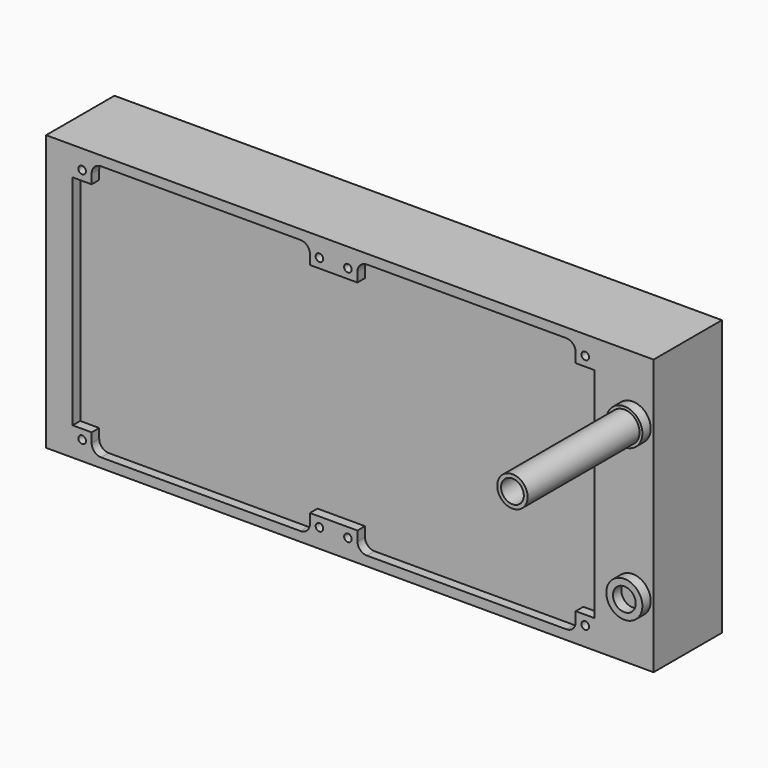
from build123d import *

# Parameters (mm, degrees)
F0_W     = 320
F0_H     = 145
F1_DEPTH = 45
F2_R     = 9.5
F2_R_2   = 6
F3_DEPTH = 5.5
F4_R     = 2
F5_DEPTH = 5
F7_R     = 8
F7_R_2   = 6
F8_DEPTH = 73.6875


# Not quite as in the source:
# - a pattern or mirror of a feature is missing from the dataset's text; its kind, count and spacing are read off the source's solid


with BuildPart() as f1:
    # F0 (on Front) → F1 (new body)
    with BuildSketch(Plane.XZ):
        with Locations((160, 0)):
            Rectangle(F0_W, F0_H)
    extrude(amount=F1_DEPTH)

    # F2 (on face) → F3 (join)
    with BuildSketch(Plane.XZ.offset(45)):
        with Locations((309, -40)):
            Circle(F2_R)
        with Locations((309, -40)):
            Circle(F2_R_2, mode=Mode.SUBTRACT)
        with Locations((309, 40)):
            Circle(F2_R)
        with Locations((309, 40)):
            Circle(F2_R_2, mode=Mode.SUBTRACT)
    extrude(amount=F3_DEPTH)

    # F4 (on face) → F5 (cut)
    with BuildSketch(Plane.XZ.offset(45)):
        with Locations((19, 62.5)):
            Circle(F4_R)
        with Locations((144, 62.5)):
            Circle(F4_R)
        with Locations((159, 62.5)):
            Circle(F4_R)
        with Locations((284, 62.5)):
            Circle(F4_R)
        with BuildLine():
            Line((24, 57.5), (14, 57.5))
            Line((14, 57.5), (14, 0))
            Line((14, 0), (14, -57.5))
            Line((14, -57.5), (24, -57.5))
            Line((24, -57.5), (24, -62.5))
            ThreePointArc((24, -62.5), (25.4644660941, -66.0355339059), (29, -67.5))
            Line((29, -67.5), (134, -67.5))
            ThreePointArc((134, -67.5), (137.5355339059, -66.0355339059), (139, -62.5))
            Line((139, -62.5), (139, -57.5))
            Line((139, -57.5), (164, -57.5))
            Line((164, -57.5), (164, -62.5))
            ThreePointArc((164, -62.5), (165.4644660941, -66.0355339059), (169, -67.5))
            Line((169, -67.5), (274, -67.5))
            ThreePointArc((274, -67.5), (277.5355339059, -66.0355339059), (279, -62.5))
            Line((279, -62.5), (279, -57.5))
            Line((279, -57.5), (289, -57.5))
            Line((289, -57.5), (289, 0))
            Line((289, 0), (289, 57.5))
            Line((289, 57.5), (279, 57.5))
            Line((279, 57.5), (279, 62.5))
            ThreePointArc((279, 62.5), (277.5355339059, 66.0355339059), (274, 67.5))
            Line((274, 67.5), (169, 67.5))
            ThreePointArc((169, 67.5), (165.4644660941, 66.0355339059), (164, 62.5))
            Line((164, 62.5), (164, 57.5))
            Line((164, 57.5), (139, 57.5))
            Line((139, 57.5), (139, 62.5))
            ThreePointArc((139, 62.5), (137.5355339059, 66.0355339059), (134, 67.5))
            Line((134, 67.5), (29, 67.5))
            ThreePointArc((29, 67.5), (25.4644660941, 66.0355339059), (24, 62.5))
            Line((24, 62.5), (24, 57.5))
        make_face()
        with Locations((284, -62.5)):
            Circle(F4_R)
        with Locations((159, -62.5)):
            Circle(F4_R)
        with Locations((144, -62.5)):
            Circle(F4_R)
        with Locations((19, -62.5)):
            Circle(F4_R)
    f5 = extrude(amount=-F5_DEPTH, mode=Mode.SUBTRACT)

    # F5_copies: F5 across plane
    add(f5.mirror(Plane.ZX.offset(-22.5)), mode=Mode.SUBTRACT)

    # F7 (on face) → F8 (join)
    with BuildSketch(Plane.XZ.offset(50.5)):
        with Locations((309, 40)):
            Circle(F7_R)
        with Locations((309, 40)):
            Circle(F7_R_2, mode=Mode.SUBTRACT)
    extrude(amount=F8_DEPTH)


solid = f1.part
